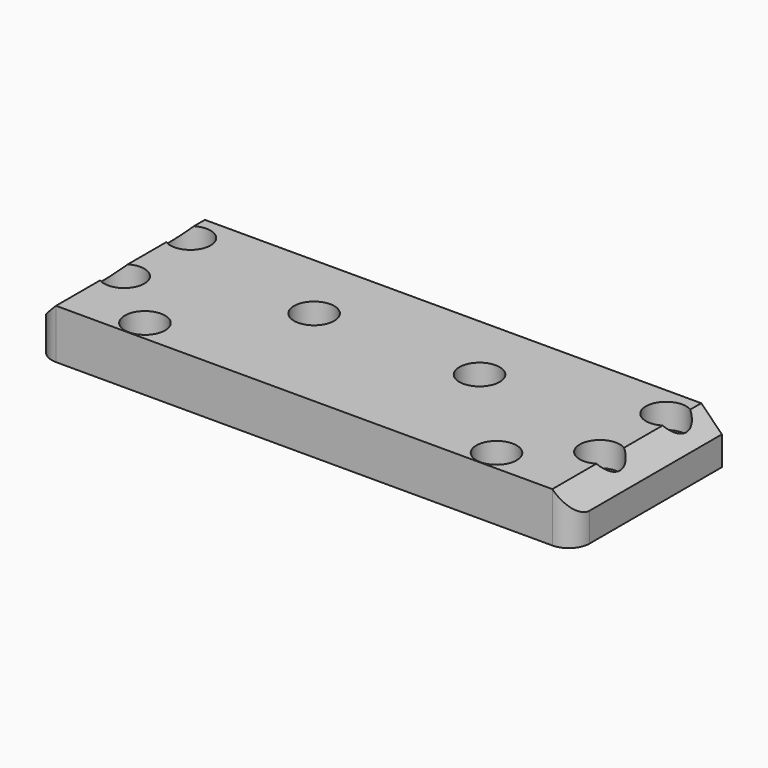
from build123d import *

# Parameters (mm, degrees)
F0_W                 = 130
F0_H                 = 45
F1_DEPTH             = 12
F2_R                 = 5
F5_D                 = 5.5
F5_CBORE_D           = 9.75
F5_CBORE_DEPTH       = 6
F5_ON_F4_D           = 5.5
F5_ON_F4_CBORE_D     = 9.75
F5_ON_F4_CBORE_DEPTH = 6
F6_T1_DEPTH          = 65.7168298797
F7_R                 = 2.75
F8_DEPTH             = 2


# Not quite as in the source:
# - a fillet or chamfer that OpenCascade refuses, or shapes differently, is made with other operations: its cross-section is extruded or revolved along the edge and cut away or added


with BuildPart() as f1:
    # F0 (on Top) → F1 (new body)
    with BuildSketch(Plane.XY):
        Rectangle(F0_W, F0_H)
    extrude(amount=F1_DEPTH)

    # F2
    f2_edges = [f1.edges().sort_by_distance(p)[0] for p in [
        (65, -22.5, 6),
        (-65, -22.5, 6),
    ]]
    fillet(f2_edges, radius=F2_R)

    # F5 (through all)
    with Locations(Plane.XY.offset(12)):
        with Locations((-57.5, -5), (-57.5, 15), (57.5, -5), (57.5, 15), (-42.5, -17.5), (42.5, -17.5)):
            CounterBoreHole(F5_D / 2, F5_CBORE_D / 2, F5_CBORE_DEPTH)

    # F5 on F4 (through all)
    with Locations(Plane.XY.offset(12)):
        with Locations((-20, 5.5), (20, 5.5)):
            CounterBoreHole(F5_ON_F4_D / 2, F5_ON_F4_CBORE_D / 2, F5_ON_F4_CBORE_DEPTH)

    # F6: chamfer of 5 on 2 edges, made by hand

    # F6_s2 → F6_t1 (cut)
    with BuildSketch(Plane.XZ.offset(-35.3584149398)):
        Polygon((-60, 12), (-65, 7), (-65, 12), align=None)
        Polygon((60, 12), (65, 7), (65, 12), align=None)
    extrude(amount=F6_T1_DEPTH, mode=Mode.SUBTRACT)

    # F7 (on face) → F8 (cut)
    with BuildSketch(Plane(origin=(0, 0, 0), x_dir=(1, 0, 0), z_dir=(0, 0, -1))):
        with BuildLine():
            Line((-18.3303027798, -22.5), (18.3303027798, -22.5))
            ThreePointArc((18.3303027798, -22.5), (25, -5.5), (18.3303027798, 11.5))
            Line((18.3303027798, 11.5), (-18.3303027798, 11.5))
            ThreePointArc((-18.3303027798, 11.5), (-25, -5.5), (-18.3303027798, -22.5))
        make_face()
        with Locations((-20, -5.5)):
            Circle(F7_R, mode=Mode.SUBTRACT)
        with Locations((20, -5.5)):
            Circle(F7_R, mode=Mode.SUBTRACT)
    extrude(amount=-F8_DEPTH, mode=Mode.SUBTRACT)


solid = f1.part
